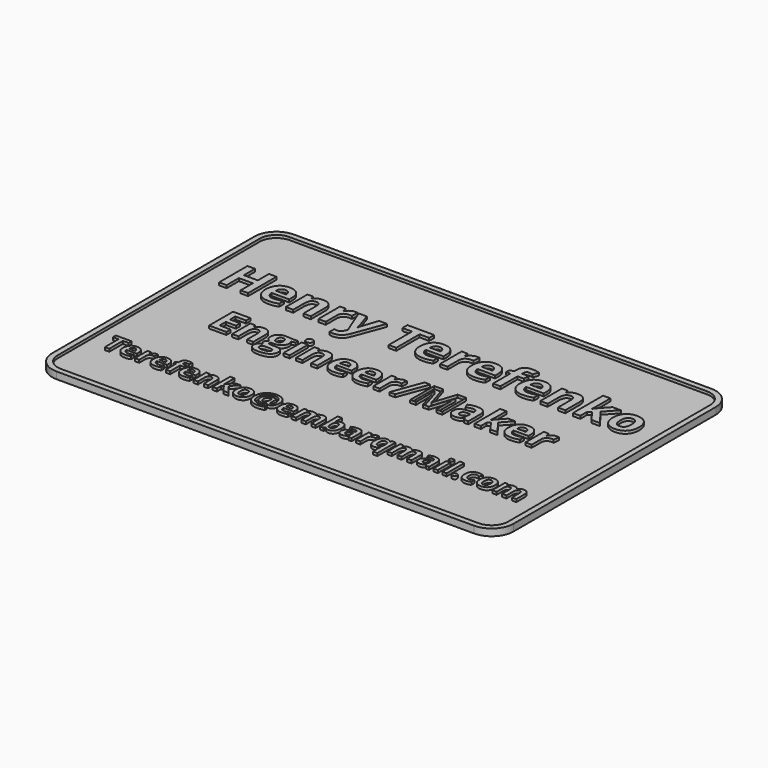
from build123d import *

# Parameters (mm, degrees)
F1_DEPTH       = 0.75
F2_TEXT_SIZE   = 9.0277777778
F2_TEXT_SIZE_2 = 7.6388888889
F2_TEXT_SIZE_3 = 5.2777777778
F3_DEPTH       = 1.25
F5_DEPTH       = 1.25


# Not quite as in the source:
# - Text() gives the source's letters only with a copy of the font that has no kerning and outlines rounded to 1/6400 em; it was checked with that copy


with BuildPart() as f1:
    # F0 (on Top) → F1 (new body)
    with BuildSketch(Plane.XY):
        with BuildLine():
            ThreePointArc((42, 23), (40.8284271247, 25.8284271247), (38, 27))
            Line((38, 27), (0, 27))
            Line((0, 27), (0, 0))
            Line((0, 0), (42, 0))
            Line((42, 0), (42, 23))
        make_face()
        with BuildLine():
            Line((0, 0), (0, 27))
            Line((0, 27), (-38, 27))
            ThreePointArc((-38, 27), (-40.8284271247, 25.8284271247), (-42, 23))
            Line((-42, 23), (-42, 0))
            Line((-42, 0), (0, 0))
        make_face()
        with BuildLine():
            Line((0, -27), (0, 0))
            Line((0, 0), (-42, 0))
            Line((-42, 0), (-42, -23))
            ThreePointArc((-42, -23), (-40.8284271247, -25.8284271247), (-38, -27))
            Line((-38, -27), (0, -27))
        make_face()
        with BuildLine():
            Line((42, 0), (0, 0))
            Line((0, 0), (0, -27))
            Line((0, -27), (38, -27))
            ThreePointArc((38, -27), (40.8284271247, -25.8284271247), (42, -23))
            Line((42, -23), (42, 0))
        make_face()
    extrude(amount=F1_DEPTH)

    # F2 (on Top) → F3 (join)
    with BuildSketch(Plane.XY):
        with Locations((-37.9132191358, 8.8586947979)):
            Text('Henry Terefenko', F2_TEXT_SIZE, font='Open Sans', font_style=FontStyle.BOLD, text_align=(TextAlign.LEFT, TextAlign.BOTTOM))
        with Locations((-30.5964860394, -2.4122077218)):
            Text('Engineer/Maker', F2_TEXT_SIZE_2, font='Open Sans', font_style=FontStyle.BOLD, text_align=(TextAlign.LEFT, TextAlign.BOTTOM))
        with Locations((-38.4643768513, -16.8459854683)):
            Text('Terefenko@embarqmail.com', F2_TEXT_SIZE_3, font='Open Sans', font_style=FontStyle.BOLD, text_align=(TextAlign.LEFT, TextAlign.BOTTOM))
    extrude(amount=F3_DEPTH)

    # F4 (on Top) → F5 (join)
    with BuildSketch(Plane.XY):
        with BuildLine():
            ThreePointArc((42, 23), (40.8284271247, 25.8284271247), (38, 27))
            Line((38, 27), (0, 27))
            Line((0, 27), (0, 26))
            Line((0, 26), (38, 26))
            ThreePointArc((38, 26), (40.1213203436, 25.1213203436), (41, 23))
            Line((41, 23), (41, 0))
            Line((41, 0), (42, 0))
            Line((42, 0), (42, 23))
        make_face()
        with BuildLine():
            Line((0, 26), (0, 27))
            Line((0, 27), (-38, 27))
            ThreePointArc((-38, 27), (-40.8284271247, 25.8284271247), (-42, 23))
            Line((-42, 23), (-42, 0))
            Line((-42, 0), (-42, -23))
            ThreePointArc((-42, -23), (-40.8284271247, -25.8284271247), (-38, -27))
            Line((-38, -27), (0, -27))
            Line((0, -27), (38, -27))
            ThreePointArc((38, -27), (40.8284271247, -25.8284271247), (42, -23))
            Line((42, -23), (42, 0))
            Line((42, 0), (41, 0))
            Line((41, 0), (41, -23))
            ThreePointArc((41, -23), (40.1213203436, -25.1213203436), (38, -26))
            Line((38, -26), (0, -26))
            Line((0, -26), (-38, -26))
            ThreePointArc((-38, -26), (-40.1213203436, -25.1213203436), (-41, -23))
            Line((-41, -23), (-41, 0))
            Line((-41, 0), (-41, 23))
            ThreePointArc((-41, 23), (-40.1213203436, 25.1213203436), (-38, 26))
            Line((-38, 26), (0, 26))
        make_face()
    extrude(amount=F5_DEPTH)


solid = f1.part
